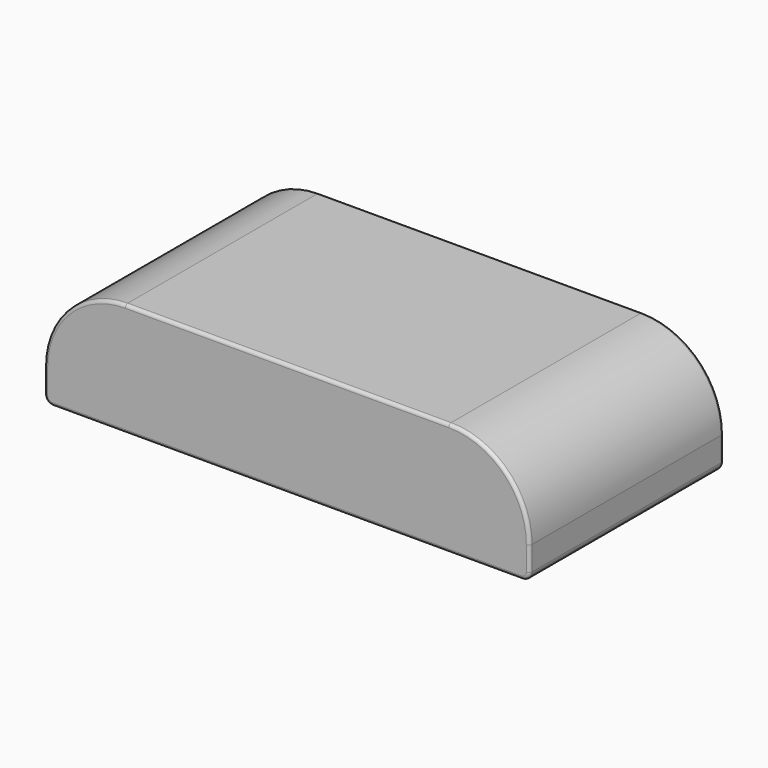
from build123d import *

# Parameters (mm, degrees)
F0_W     = 300
F0_H     = 150
F1_DEPTH = 70
F2_R     = 50
F3_R     = 5
F4_R     = 2


with BuildPart() as f1:
    # F0 (on Top) → F1 (new body)
    with BuildSketch(Plane.XY):
        with Locations((150, 78.7498958572)):
            Rectangle(F0_W, F0_H)
    extrude(amount=F1_DEPTH)

    # F2
    f2_edges = [f1.edges().sort_by_distance(p)[0] for p in [
        (0, 78.749896, 70),
        (300, 78.749896, 70),
    ]]
    fillet(f2_edges, radius=F2_R)

    # F3
    f3_edges = [f1.edges().sort_by_distance(p)[0] for p in [
        (0, 78.749896, 0),
        (300, 78.749896, 0),
    ]]
    fillet(f3_edges, radius=F3_R)

    # F4
    f4_edges = [f1.edges().sort_by_distance(p)[0] for p in [
        (150, 3.749896, 70),
        (150, 153.749896, 70),
        (150, 3.749896, 0),
        (150, 153.749896, 0),
        (300, 3.749896, 12.5),
        (300, 153.749896, 12.5),
        (0, 3.749896, 12.5),
        (1.464466, 3.749896, 1.464466),
        (14.644661, 3.749896, 55.355339),
        (298.535534, 3.749896, 1.464466),
        (285.355339, 3.749896, 55.355339),
        (298.535534, 153.749896, 1.464466),
        (285.355339, 153.749896, 55.355339),
        (1.464466, 153.749896, 1.464466),
        (14.644661, 153.749896, 55.355339),
        (0, 153.749896, 12.5),
    ]]
    fillet(f4_edges, radius=F4_R)


solid = f1.part
